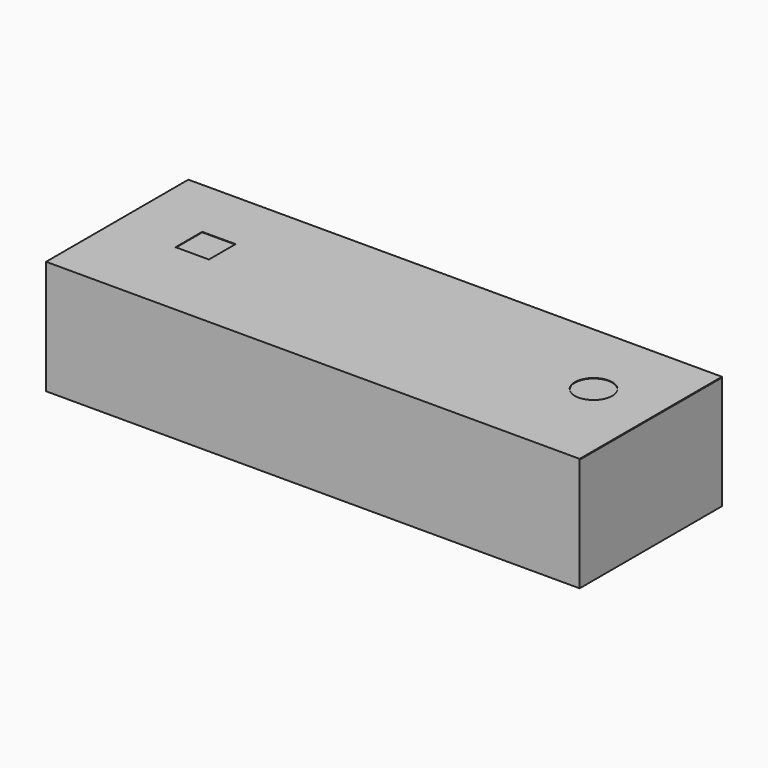
from build123d import *

# Parameters (mm, degrees)
F1_DEPTH = 209.55
F2_W     = 26.19375
F2_H     = 26.19375
F3_DEPTH = 0.4064


# Not quite as in the source:
# - the dataset's text gives a spline's control points without its knots; the knots are read off the source's solid


with BuildPart() as f1:
    # F0 (on Right) → F1 (new body, symmetric)
    with BuildSketch(Plane.YZ):
        Polygon((-139.7, 0), (0, 0), (0, 88.9), (-139.2936, 88.9), (-139.2936, 89.154), (0, 89.154), (0, 89.5604), (-139.7, 89.5604), align=None)
    extrude(amount=F1_DEPTH, both=True)

    # F2 (on face) → F3 (cut, through all)
    with BuildSketch(Plane.XY.offset(89.5604)):
        with Locations((-146.5180454731, -61.8854577733)):
            Rectangle(F2_W, F2_H)
        with BuildLine():
            add(Edge.make_bspline(
                [(168.6654745269, -51.5019377733), (165.9469379269, -48.7836043733), (162.1263207269, -47.2010827733), (158.2819545269, -47.2010827733)],
                knots=[7, 7, 7, 7, 8, 8, 8, 8], degree=3))
            add(Edge.make_bspline(
                [(158.2819545269, -47.2010827733), (154.4375629269, -47.2010827733), (150.6169457269, -48.7836043733), (147.8987647269, -51.5019377733)],
                knots=[0, 0, 0, 0, 1, 1, 1, 1], degree=3))
            add(Edge.make_bspline(
                [(147.8987647269, -51.5019377733), (145.1802535269, -54.2204743733), (143.5975795269, -58.0410915733), (143.5975795269, -61.8854577733), (143.5975795269, -65.7298493733), (145.1802535269, -69.5504665733), (147.8987647269, -72.2689777733)],
                knots=[1, 1, 1, 1, 2, 2, 2, 3, 3, 3, 3], degree=3))
            add(Edge.make_bspline(
                [(147.8987647269, -72.2689777733), (150.6169457269, -74.9873365733), (154.4375629269, -76.5698327733), (158.2819545269, -76.5698327733), (162.1263207269, -76.5698327733), (165.9469379269, -74.9873365733), (168.6654745269, -72.2689777733)],
                knots=[3, 3, 3, 3, 4, 4, 4, 5, 5, 5, 5], degree=3))
            add(Edge.make_bspline(
                [(168.6654745269, -72.2689777733), (171.3839857269, -69.5504665733), (172.9663295269, -65.7298493733), (172.9663295269, -61.8854577733), (172.9663295269, -58.0410915733), (171.3839857269, -54.2204743733), (168.6654745269, -51.5019377733)],
                knots=[5, 5, 5, 5, 6, 6, 6, 7, 7, 7, 7], degree=3))
        make_face()
    extrude(amount=-F3_DEPTH, mode=Mode.SUBTRACT)


solid = f1.part
